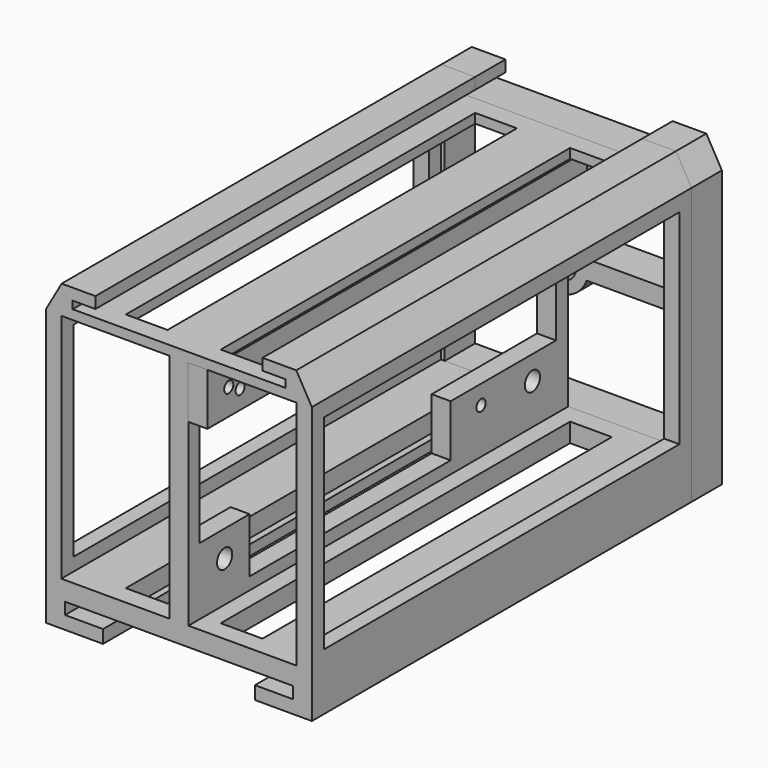
from build123d import *

# Parameters (mm, degrees)
F1_DEPTH       = 125
F2_W           = 28.5
F2_H           = 60.95
F3_DEPTH       = 152.27041
F4_W           = 117
F4_H           = 53.8040182785
F5_DEPTH       = 25
F8_R           = 1.5
F8_R_2         = 2.5
F9_DEPTH       = 5
F10_R          = 1.5
F11_DEPTH      = 5
F11_DEPTH_BACK = 0.1
F13_DEPTH      = 10
F14_R          = 4.7625
F15_DEPTH      = 12
F16_R          = 1
F17_DEPTH      = 25
F18_W          = 11
F18_H          = 115
F19_DEPTH      = 106.67049


# Not quite as in the source:
# - a feature names something its author has since deleted; it is built from what else it names


with BuildPart() as f1:
    # F0 (on Front) → F1 (new body)
    with BuildSketch(Plane.XZ):
        Polygon((-44.2135502246, 32.3922252908), (-44.2135502246, 35.3922252908), (-53.1108938158, 35.3922252908), (-57.2135502246, 28.1962435693), (-57.2135502246, 25.3922252908), (-57.2135502246, -44.6077747092), (-42.2135502246, -44.6077747092), (-42.2135502246, -41.1577747092), (-52.2135502246, -41.1577747092), (-52.2135502246, -38.0577747092), (-22.2135502246, -38.0577747092), (7.7864497754, -38.0577747092), (7.7864497754, -41.1577747092), (-2.2135502246, -41.1577747092), (-2.2135502246, -44.6077747092), (12.7864497754, -44.6077747092), (12.7864497754, 25.3922252908), (12.7864497754, 28.1962435693), (8.6837933666, 35.3922252908), (-0.2135502246, 35.3922252908), (-0.2135502246, 32.3922252908), (5.7864497754, 32.3922252908), (5.7864497754, 30.3922252908), (-22.2135502246, 30.3922252908), (-50.2135502246, 30.3922252908), (-50.2135502246, 32.3922252908), align=None)
    extrude(amount=F1_DEPTH)

    # F2 (on face) → F3 (cut)
    with BuildSketch(Plane(origin=(0, 0, 0), x_dir=(-1, 0, 0), z_dir=(0, 1, 0))):
        with Locations((5.4635502246, -2.5827747092)):
            Rectangle(F2_W, F2_H)
        with Locations((38.9635502246, -2.5827747092)):
            Rectangle(F2_W, F2_H)
    extrude(amount=-F3_DEPTH, mode=Mode.SUBTRACT)

    # F4 (on face) → F5 (cut)
    with BuildSketch(Plane(origin=(-57.2135502246, 0, 0), x_dir=(0, -1, 0), z_dir=(-1, 0, 0))):
        with Locations((62.5, -2.70576557)):
            Rectangle(F4_W, F4_H)
    f5 = extrude(amount=-F5_DEPTH, mode=Mode.SUBTRACT)

    # F7: F5 across plane
    add(f5.mirror(Plane(origin=(-22.2135502246, -62.5, -2.5827747092), x_dir=(0, 1, 0), z_dir=(1, 0, 0))), mode=Mode.SUBTRACT)

    # F8 (on face) → F9 (cut, through all)
    with BuildSketch(Plane(origin=(-24.7135502246, 0, 0), x_dir=(0, -1, 0), z_dir=(-1, 0, 0))):
        Polygon((18.6793928742, 14.8922252908), (18.6793928742, 24.1962435693), (14, 24.1962435693), (14, 14.8922252908), (4, 14.8922252908), (4, -16.1077747092), (18.6793928742, -16.1077747092), (38.6793928742, -16.1077747092), (38.6793928742, -29.8098996476), (104.8905849457, -29.8098996476), (104.8905849457, -15.3639111668), (121.439190805, -15.3935970739), (121.439190805, 14.8922252908), (111.439190805, 14.8922252908), (111.439190805, 24.1962435693), (104.6793928742, 24.1962435693), (104.6793928742, 14.8922252908), (84.6793928742, 14.8922252908), (84.6793928742, 24.1592433304), (72.1670018911, 24.1592433304), (72.1670018911, 11.4058125764), (52.097171545, 11.4058125764), (52.097171545, 24.1592433304), (38.6793928742, 24.1592433304), (38.6793928742, 14.8922252908), align=None)
        with Locations((9, 19.54423443)):
            Circle(F8_R)
        with Locations((28.6793928742, 19.8922252908)):
            Circle(F8_R)
        with Locations((94.6793928742, 19.8922252908)):
            Circle(F8_R)
        with Locations((28.6793928742, -21.1077747092)):
            Circle(F8_R)
        with Locations((117.9832443595, 21.0658144206)):
            Circle(F8_R)
        with Locations((62.5, 17.3922252908)):
            Circle(F8_R_2)
        with Locations((11.7614362389, -22.3910976201)):
            Circle(F8_R_2)
        with Locations((113.0883896302, -22.341915994)):
            Circle(F8_R_2)
    extrude(amount=-F9_DEPTH, mode=Mode.SUBTRACT)

    # F18 (on face) → F19 (cut)
    with BuildSketch(Plane.XY.offset(30.3922252908)):
        with Locations((-34.7135502246, -62.5)):
            Rectangle(F18_W, F18_H)
        with Locations((-9.7135502246, -62.5)):
            Rectangle(F18_W, F18_H)
    extrude(amount=-F19_DEPTH, mode=Mode.SUBTRACT)


with BuildPart() as f11:
    # F10 (on face) → F11 (new body, two sides)
    with BuildSketch(Plane.YZ.offset(-19.7135502246)) as f11_sk:
        with BuildLine():
            Line((-125, 14.1962435693), (-121.8479664919, 14.1962435693))
            Line((-121.8479664919, 14.1962435693), (-121.439190805, 14.1962435693))
            Line((-121.439190805, 14.1962435693), (-121.439190805, 14.8922252908))
            Line((-121.439190805, 14.8922252908), (-111.439190805, 14.8922252908))
            Line((-111.439190805, 14.8922252908), (-111.439190805, 24.1962435693))
            Line((-111.439190805, 24.1962435693), (-104.6793928742, 24.1962435693))
            Line((-104.6793928742, 24.1962435693), (-104.6793928742, 20.6223889284))
            ThreePointArc((-104.6793928742, 20.6223889284), (-103.333413762, 20.4101862259), (-102.7145171762, 19.1962435693))
            ThreePointArc((-102.7145171762, 19.1962435693), (-103.333413762, 17.9823009126), (-104.6793928742, 17.7700982101))
            Line((-104.6793928742, 17.7700982101), (-104.6793928742, 14.8922252908))
            Line((-104.6793928742, 14.8922252908), (-84.6793928742, 14.8922252908))
            Line((-84.6793928742, 14.8922252908), (-84.6793928742, 17.7700982101))
            ThreePointArc((-84.6793928742, 17.7700982101), (-85.7145171762, 19.1962435693), (-84.6793928742, 20.6223889284))
            Line((-84.6793928742, 20.6223889284), (-84.6793928742, 24.1592433304))
            Line((-84.6793928742, 24.1592433304), (-72.1670018911, 24.1592433304))
            Line((-72.1670018911, 24.1592433304), (-72.1670018911, 14.1962435693))
            Line((-72.1670018911, 14.1962435693), (-52.097171545, 14.1962435693))
            Line((-52.097171545, 14.1962435693), (-52.097171545, 24.1592433304))
            Line((-52.097171545, 24.1592433304), (-38.6793928742, 24.1592433304))
            Line((-38.6793928742, 24.1592433304), (-38.6793928742, 14.8922252908))
            Line((-38.6793928742, 14.8922252908), (-18.6793928742, 14.8922252908))
            Line((-18.6793928742, 14.8922252908), (-18.6793928742, 24.1962435693))
            Line((-18.6793928742, 24.1962435693), (-14, 24.1962435693))
            Line((-14, 24.1962435693), (-14, 20.6808251201))
            ThreePointArc((-14, 20.6808251201), (-13.0805472109, 20.1781356804), (-12.7145171762, 19.1962435693))
            ThreePointArc((-12.7145171762, 19.1962435693), (-13.0805472109, 18.2143514581), (-14, 17.7116620184))
            Line((-14, 17.7116620184), (-14, 14.8922252908))
            Line((-14, 14.8922252908), (-4, 14.8922252908))
            Line((-4, 14.8922252908), (-4, 14.1962435693))
            Line((-4, 14.1962435693), (0, 14.1962435693))
            Line((0, 14.1962435693), (0, 27.8922252908))
            Line((0, 27.8922252908), (-125, 27.8922252908))
            Line((-125, 27.8922252908), (-125, 14.1962435693))
        make_face()
        with Locations((-114.2145171762, 19.1962435693)):
            Circle(F10_R, mode=Mode.SUBTRACT)
        with BuildLine():
            ThreePointArc((-93.249140038, 20.3443058416), (-92.8547257018, 19.829463236), (-92.7145171762, 19.1962435693))
            ThreePointArc((-92.7145171762, 19.1962435693), (-93.9858025662, 17.7137829029), (-95.6447700124, 18.7441630185))
            ThreePointArc((-95.6447700124, 18.7441630185), (-95.5125444914, 21.1395658148), (-93.249140038, 20.3443058416))
        make_face(mode=Mode.SUBTRACT)
        with Locations((-117.9832443595, 21.0658144206)):
            Circle(F10_R, mode=Mode.SUBTRACT)
        with BuildLine():
            ThreePointArc((-64.9501434301, 17.8890121382), (-65.2478630448, 20.2835320846), (-62.8715762211, 19.8644573009))
            ThreePointArc((-62.8715762211, 19.8644573009), (-60.8688869679, 19.2868150291), (-60, 17.3922252908))
            ThreePointArc((-60, 17.3922252908), (-62.7496411671, 14.9047206601), (-64.9501434301, 17.8890121382))
        make_face(mode=Mode.SUBTRACT)
        with Locations((-54.2145171762, 19.1962435693)):
            Circle(F10_R, mode=Mode.SUBTRACT)
        with Locations((-34.2145171762, 19.1962435693)):
            Circle(F10_R, mode=Mode.SUBTRACT)
        with Locations((-28.6793928742, 19.8922252908)):
            Circle(F10_R, mode=Mode.SUBTRACT)
        with Locations((-24.2145171762, 19.1962435693)):
            Circle(F10_R, mode=Mode.SUBTRACT)
        with Locations((-9, 19.54423443)):
            Circle(F10_R, mode=Mode.SUBTRACT)
        with BuildLine():
            Line((-121.439190805, 14.8922252908), (-121.439190805, 14.1962435693))
            Line((-121.439190805, 14.1962435693), (-72.1670018911, 14.1962435693))
            Line((-72.1670018911, 14.1962435693), (-72.1670018911, 24.1592433304))
            Line((-72.1670018911, 24.1592433304), (-84.6793928742, 24.1592433304))
            Line((-84.6793928742, 24.1592433304), (-84.6793928742, 20.6223889284))
            ThreePointArc((-84.6793928742, 20.6223889284), (-83.333413762, 20.4101862259), (-82.7145171762, 19.1962435693))
            ThreePointArc((-82.7145171762, 19.1962435693), (-83.333413762, 17.9823009126), (-84.6793928742, 17.7700982101))
            Line((-84.6793928742, 17.7700982101), (-84.6793928742, 14.8922252908))
            Line((-84.6793928742, 14.8922252908), (-104.6793928742, 14.8922252908))
            Line((-104.6793928742, 14.8922252908), (-104.6793928742, 17.7700982101))
            ThreePointArc((-104.6793928742, 17.7700982101), (-105.7145171762, 19.1962435693), (-104.6793928742, 20.6223889284))
            Line((-104.6793928742, 20.6223889284), (-104.6793928742, 24.1962435693))
            Line((-104.6793928742, 24.1962435693), (-111.439190805, 24.1962435693))
            Line((-111.439190805, 24.1962435693), (-111.439190805, 14.8922252908))
            Line((-111.439190805, 14.8922252908), (-121.439190805, 14.8922252908))
        make_face()
        with Locations((-74.2145171762, 19.1962435693)):
            Circle(F10_R, mode=Mode.SUBTRACT)
        with BuildLine():
            Line((-52.097171545, 24.1592433304), (-52.097171545, 14.1962435693))
            Line((-52.097171545, 14.1962435693), (-4, 14.1962435693))
            Line((-4, 14.1962435693), (-4, 14.8922252908))
            Line((-4, 14.8922252908), (-14, 14.8922252908))
            Line((-14, 14.8922252908), (-14, 17.7116620184))
            ThreePointArc((-14, 17.7116620184), (-15.7145171762, 19.1962435693), (-14, 20.6808251201))
            Line((-14, 20.6808251201), (-14, 24.1962435693))
            Line((-14, 24.1962435693), (-18.6793928742, 24.1962435693))
            Line((-18.6793928742, 24.1962435693), (-18.6793928742, 14.8922252908))
            Line((-18.6793928742, 14.8922252908), (-38.6793928742, 14.8922252908))
            Line((-38.6793928742, 14.8922252908), (-38.6793928742, 24.1592433304))
            Line((-38.6793928742, 24.1592433304), (-52.097171545, 24.1592433304))
        make_face()
        with Locations((-44.2145171762, 19.1962435693)):
            Circle(F10_R, mode=Mode.SUBTRACT)
        with BuildLine():
            ThreePointArc((-62.8715762211, 19.8644573009), (-62.7543097538, 19.5394552877), (-62.7145171762, 19.1962435693))
            ThreePointArc((-62.7145171762, 19.1962435693), (-63.4573644112, 17.9013614547), (-64.9501434301, 17.8890121382))
            ThreePointArc((-64.9501434301, 17.8890121382), (-62.7496411671, 14.9047206601), (-60, 17.3922252908))
            ThreePointArc((-60, 17.3922252908), (-60.8688869679, 19.2868150291), (-62.8715762211, 19.8644573009))
        make_face()
    extrude(amount=F11_DEPTH)
    extrude(f11_sk.sketch, amount=-F11_DEPTH_BACK)


with BuildPart() as f13:
    # F12 (on face) → F13 (new body)
    with BuildSketch(Plane(origin=(0, 0, 0), x_dir=(-1, 0, 0), z_dir=(0, 1, 0))):
        Polygon((0.2135502246, 32.3922252908), (0.2135502246, 35.3922252908), (-8.6837933666, 35.3922252908), (-12.7864497754, 28.1962435693), (-12.7864497754, -44.6077747092), (2.2135502246, -44.6077747092), (2.2135502246, -41.1577747092), (-7.7864497754, -41.1577747092), (-7.7864497754, -38.0577747092), (52.2135502246, -38.0577747092), (52.2135502246, -41.1577747092), (42.2135502246, -41.1577747092), (42.2135502246, -44.6077747092), (57.2135502246, -44.6077747092), (57.2135502246, 28.1962435693), (53.1108938158, 35.3922252908), (44.2135502246, 35.3922252908), (44.2135502246, 32.3922252908), (50.2135502246, 32.3922252908), (50.2135502246, 30.3922252908), (-5.7864497754, 30.3922252908), (-5.7864497754, 32.3922252908), align=None)
    extrude(amount=F13_DEPTH)

    # F14 (on face) → F15 (cut)
    with BuildSketch(Plane(origin=(0, 10, 0), x_dir=(-1, 0, 0), z_dir=(0, 1, 0))):
        with Locations((22.2135502246, 0.2297252908)):
            Circle(F14_R)
        with BuildLine():
            ThreePointArc((14.864645119, 2.7297252908), (16.7246338356, 5.7186416798), (19.7135502246, 7.5786303963))
            Line((19.7135502246, 7.5786303963), (19.7135502246, 25.3922252908))
            Line((19.7135502246, 25.3922252908), (-7.7864497754, 25.3922252908))
            Line((-7.7864497754, 25.3922252908), (-7.7864497754, 2.7297252908))
            Line((-7.7864497754, 2.7297252908), (14.864645119, 2.7297252908))
        make_face()
        with BuildLine():
            ThreePointArc((24.7135502246, 7.5786303963), (27.7024666135, 5.7186416798), (29.5624553301, 2.7297252908))
            Line((29.5624553301, 2.7297252908), (52.2135502246, 2.7297252908))
            Line((52.2135502246, 2.7297252908), (52.2135502246, 25.3922252908))
            Line((52.2135502246, 25.3922252908), (24.7135502246, 25.3922252908))
            Line((24.7135502246, 25.3922252908), (24.7135502246, 7.5786303963))
        make_face()
        with BuildLine():
            Line((52.2135502246, -2.2702747092), (29.5624553301, -2.2702747092))
            ThreePointArc((29.5624553301, -2.2702747092), (22.2135502246, -7.5327747092), (14.864645119, -2.2702747092))
            Line((14.864645119, -2.2702747092), (-7.7864497754, -2.2702747092))
            Line((-7.7864497754, -2.2702747092), (-7.7864497754, -33.0577747092))
            Line((-7.7864497754, -33.0577747092), (52.2135502246, -33.0577747092))
            Line((52.2135502246, -33.0577747092), (52.2135502246, -2.2702747092))
        make_face()
    extrude(amount=-F15_DEPTH, mode=Mode.SUBTRACT)

    # F16 (on face) → F17 (cut)
    with BuildSketch(Plane(origin=(0, 10, 0), x_dir=(-1, 0, 0), z_dir=(0, 1, 0))):
        with Locations((-9.419497017, 27.9174055904)):
            Circle(F16_R)
        with Locations((-10.3425895795, -35.4378335178)):
            Circle(F16_R)
        with Locations((54.4995330274, -35.4378335178)):
            Circle(F16_R)
        with Locations((53.0972331762, 27.9174055904)):
            Circle(F16_R)
    extrude(amount=-F17_DEPTH, mode=Mode.SUBTRACT)


solid = Compound([f1.part, f11.part, f13.part])
